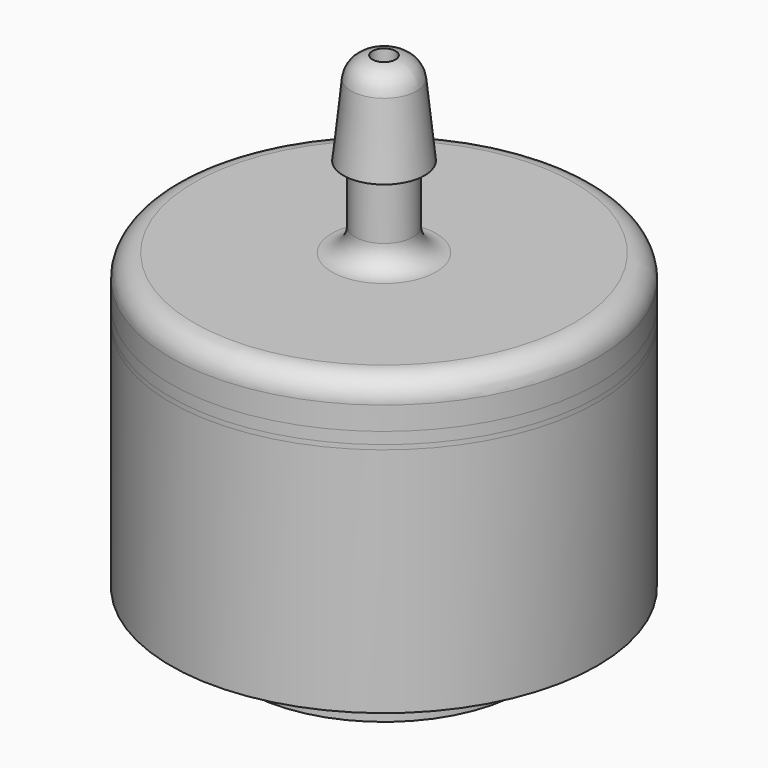
from build123d import *

# Parameters (mm, degrees)
F0_R      = 6
F0_R_2    = 3.1
F0_R_3    = 0.5
F1_DEPTH  = 2
F2_R      = 2.75
F3_DEPTH  = 0.2
F4_R      = 3.1
F4_R_2    = 2.7
F5_DEPTH  = 1
F4_R_3    = 6
F6_DEPTH  = 10
F8_R      = 6
F8_R_2    = 0.5
F9_DEPTH  = 0.2
F8_R_3    = 9.2
F8_R_4    = 6.2
F10_DEPTH = 10
F11_DEPTH = 0.2
F12_R     = 9.2
F12_R_2   = 6.2
F13_DEPTH = 0.5
F14_R     = 9.2
F15_DEPTH = 2
F16_R     = 1.25
F17_DEPTH = 3.5
F18_R     = 1.75
F18_R_2   = 1.25
F19_DEPTH = 4
F19_TAPER = 6
F20_R     = 0.5
F21_DEPTH = 25
F23_R     = 0.5


# Not quite as in the source:
# - a fillet or chamfer that OpenCascade refuses, or shapes differently, is made with other operations: its cross-section is extruded or revolved along the edge and cut away or added
# - a feature names something its author has since deleted; it is built from what else it names


with BuildPart() as f1:
    # F0 (on Top) → F1 (new body)
    with BuildSketch(Plane.XY):
        Circle(F0_R)
        Circle(F0_R_2, mode=Mode.SUBTRACT)
        Circle(F0_R_2)
        with Locations((-1.7320508076, -1)):
            Circle(F0_R_3, mode=Mode.SUBTRACT)
        with Locations((0, -2)):
            Circle(F0_R_3, mode=Mode.SUBTRACT)
        with Locations((1.7320508076, -1)):
            Circle(F0_R_3, mode=Mode.SUBTRACT)
        with Locations((-1.7320508076, 1)):
            Circle(F0_R_3, mode=Mode.SUBTRACT)
        Circle(F0_R_3, mode=Mode.SUBTRACT)
        with Locations((1.7320508076, 1)):
            Circle(F0_R_3, mode=Mode.SUBTRACT)
        with Locations((0, 2)):
            Circle(F0_R_3, mode=Mode.SUBTRACT)
    extrude(amount=-F1_DEPTH)

    # F2 (on face) → F3 (cut)
    with BuildSketch(Plane.XY):
        Circle(F2_R)
        with BuildLine():
            ThreePointArc((2.1364027102, 0.7058919606), (2.221419152, 0.3574869943), (2.25, 0))
            ThreePointArc((2.25, 0), (2.221419152, -0.3574869943), (2.1364027102, -0.7058919606))
            ThreePointArc((2.1364027102, -0.7058919606), (2.2075379006, -0.845364867), (2.2320508076, -1))
            ThreePointArc((2.2320508076, -1), (2.0665171428, -1.3716615), (1.6795217253, -1.4972330394))
            ThreePointArc((1.6795217253, -1.4972330394), (1.125, -1.9485571585), (0.4568809849, -2.203125))
            ThreePointArc((0.4568809849, -2.203125), (0, -2.5), (-0.4568809849, -2.203125))
            ThreePointArc((-0.4568809849, -2.203125), (-1.125, -1.9485571585), (-1.6795217253, -1.4972330394))
            ThreePointArc((-1.6795217253, -1.4972330394), (-2.1650635095, -1.25), (-2.1364027102, -0.7058919606))
            ThreePointArc((-2.1364027102, -0.7058919606), (-2.25, 0), (-2.1364027102, 0.7058919606))
            ThreePointArc((-2.1364027102, 0.7058919606), (-2.1650635095, 1.25), (-1.6795217253, 1.4972330394))
            ThreePointArc((-1.6795217253, 1.4972330394), (-1.125, 1.9485571585), (-0.4568809849, 2.203125))
            ThreePointArc((-0.4568809849, 2.203125), (0, 2.5), (0.4568809849, 2.203125))
            ThreePointArc((0.4568809849, 2.203125), (1.125, 1.9485571585), (1.6795217253, 1.4972330394))
            ThreePointArc((1.6795217253, 1.4972330394), (2.0665171428, 1.3716615), (2.2320508076, 1))
            ThreePointArc((2.2320508076, 1), (2.2075379006, 0.845364867), (2.1364027102, 0.7058919606))
        make_face(mode=Mode.SUBTRACT)
    extrude(amount=-F3_DEPTH, mode=Mode.SUBTRACT)

    # F4 (on face) → F5 (join)
    with BuildSketch(Plane(origin=(0, 0, -2), x_dir=(1, 0, 0), z_dir=(0, 0, -1))):
        Circle(F4_R)
        Circle(F4_R_2, mode=Mode.SUBTRACT)
    extrude(amount=F5_DEPTH)

    # F4 (on face) → F6 (join)
    with BuildSketch(Plane(origin=(0, 0, -2), x_dir=(1, 0, 0), z_dir=(0, 0, -1))):
        Circle(F4_R_3)
        Circle(F4_R, mode=Mode.SUBTRACT)
    extrude(amount=F6_DEPTH)

    # F23
    f23_edges = [f1.edges().sort_by_distance(p)[0] for p in [
        (-6, 0, 0),
    ]]
    fillet(f23_edges, radius=F23_R)


with BuildPart() as f9:
    # F8 (on offset) → F9 (new body)
    with BuildSketch(Plane.XY):
        Circle(F8_R)
        with Locations((-1.7320508076, -1)):
            Circle(F8_R_2, mode=Mode.SUBTRACT)
        with Locations((0, -2)):
            Circle(F8_R_2, mode=Mode.SUBTRACT)
        with Locations((1.7320508076, -1)):
            Circle(F8_R_2, mode=Mode.SUBTRACT)
        with Locations((-1.7320508076, 1)):
            Circle(F8_R_2, mode=Mode.SUBTRACT)
        Circle(F8_R_2, mode=Mode.SUBTRACT)
        with Locations((1.7320508076, 1)):
            Circle(F8_R_2, mode=Mode.SUBTRACT)
        with Locations((0, 2)):
            Circle(F8_R_2, mode=Mode.SUBTRACT)
        with Locations((-1.7320508076, 1)):
            Circle(F8_R_2)
        with Locations((0, 2)):
            Circle(F8_R_2)
        with Locations((1.7320508076, 1)):
            Circle(F8_R_2)
        with Locations((1.7320508076, -1)):
            Circle(F8_R_2)
        with Locations((0, -2)):
            Circle(F8_R_2)
        with Locations((-1.7320508076, -1)):
            Circle(F8_R_2)
        Circle(F8_R_2)
    extrude(amount=F9_DEPTH)


with BuildPart() as f10:
    # F8 (on offset) → F10 (new body)
    with BuildSketch(Plane.XY):
        Circle(F8_R_3)
        Circle(F8_R_4, mode=Mode.SUBTRACT)
    extrude(amount=-F10_DEPTH)

    # F11 (add): a face of the model
    f11_faces = [f10.faces().sort_by_distance(p)[0] for p in [
        (-8.9397847045, 0, 0),
    ]]
    extrude(f11_faces, amount=F11_DEPTH)

    # F12 (on face) → F13 (join)
    with BuildSketch(Plane.XY.offset(0.2)):
        Circle(F12_R)
        Circle(F12_R_2, mode=Mode.SUBTRACT)
        Circle(F12_R_2)
        with BuildLine():
            ThreePointArc((-3, 0), (-2.7071067812, 0.7071067812), (-2, 1))
            Line((-2, 1), (-1, 1))
            Line((-1, 1), (-1, 2))
            ThreePointArc((-1, 2), (-0.7071067812, 2.7071067812), (0, 3))
            ThreePointArc((0, 3), (0.7071067812, 2.7071067812), (1, 2))
            Line((1, 2), (1, 1))
            Line((1, 1), (2, 1))
            ThreePointArc((2, 1), (2.7071067812, 0.7071067812), (3, 0))
            ThreePointArc((3, 0), (2.7071067812, -0.7071067812), (2, -1))
            Line((2, -1), (1, -1))
            Line((1, -1), (1, -2))
            ThreePointArc((1, -2), (0.7071067812, -2.7071067812), (0, -3))
            ThreePointArc((0, -3), (-0.7071067812, -2.7071067812), (-1, -2))
            Line((-1, -2), (-1, -1))
            Line((-1, -1), (-2, -1))
            ThreePointArc((-2, -1), (-2.7071067812, -0.7071067812), (-3, 0))
        make_face(mode=Mode.SUBTRACT)
    extrude(amount=F13_DEPTH)

    # F14 (on face) → F15 (join)
    with BuildSketch(Plane.XY.offset(0.7)):
        Circle(F14_R)
        with BuildLine():
            ThreePointArc((1, -2), (0, -3), (-1, -2))
            Line((-1, -2), (-1, -1))
            Line((-1, -1), (-2, -1))
            ThreePointArc((-2, -1), (-3, 0), (-2, 1))
            Line((-2, 1), (-1, 1))
            Line((-1, 1), (-1, 2))
            ThreePointArc((-1, 2), (0, 3), (1, 2))
            Line((1, 2), (1, 1))
            Line((1, 1), (2, 1))
            ThreePointArc((2, 1), (3, 0), (2, -1))
            Line((2, -1), (1, -1))
            Line((1, -1), (1, -2))
        make_face(mode=Mode.SUBTRACT)
        with BuildLine():
            Line((-1, -1), (-1, -2))
            ThreePointArc((-1, -2), (0, -3), (1, -2))
            Line((1, -2), (1, -1))
            Line((1, -1), (2, -1))
            ThreePointArc((2, -1), (3, 0), (2, 1))
            Line((2, 1), (1, 1))
            Line((1, 1), (1, 2))
            ThreePointArc((1, 2), (0, 3), (-1, 2))
            Line((-1, 2), (-1, 1))
            Line((-1, 1), (-2, 1))
            ThreePointArc((-2, 1), (-3, 0), (-2, -1))
            Line((-2, -1), (-1, -1))
        make_face()
    extrude(amount=F15_DEPTH)

    # F16 (on face) → F17 (join)
    with BuildSketch(Plane.XY.offset(2.7)):
        Circle(F16_R)
    extrude(amount=F17_DEPTH)

    # F18 (on face) → F19 (join)
    with BuildSketch(Plane.XY.offset(6.2)):
        Circle(F18_R)
        Circle(F18_R_2, mode=Mode.SUBTRACT)
        Circle(F18_R_2)
    extrude(amount=F19_DEPTH, taper=F19_TAPER)

    # F20 (on face) → F21 (cut)
    with BuildSketch(Plane.XY.offset(10.2)):
        Circle(F20_R)
    extrude(amount=-F21_DEPTH, mode=Mode.SUBTRACT)

    # F22: fillet of radius 1 on 3 edges, made by hand

    # F22_s1 → F22_t2 (revolve)
    with BuildSketch(Plane.XZ):
        with BuildLine():
            ThreePointArc((1.25, 3.7), (1.5428932188, 2.9928932188), (2.25, 2.7))
            Line((2.25, 2.7), (1.25, 2.7))
            Line((1.25, 2.7), (1.25, 3.7))
        make_face()
    revolve(axis=Axis((0, 0, 2.7), (0, 0, 1)))

    # F22_s3 → F22_t4 (revolve, cut)
    with BuildSketch(Plane.XZ):
        with BuildLine():
            ThreePointArc((1.4234350097, 9.3070583361), (1.1240510304, 9.9214062722), (0.5, 10.2))
            Line((0.5, 10.2), (1.3295830589, 10.2))
            Line((1.3295830589, 10.2), (1.4234350097, 9.3070583361))
        make_face()
    revolve(axis=Axis((0, 0, 10.2), (0, 0, -1)), mode=Mode.SUBTRACT)

    # F22_s5 → F22_t6 (revolve, cut)
    with BuildSketch(Plane.XZ):
        with BuildLine():
            ThreePointArc((8.2, 2.7), (8.9071067812, 2.4071067812), (9.2, 1.7))
            Line((9.2, 1.7), (9.2, 2.7))
            Line((9.2, 2.7), (8.2, 2.7))
        make_face()
    revolve(axis=Axis((0, 0, 2.7), (0, 0, 1)), mode=Mode.SUBTRACT)


solid = Compound([f1.part, f9.part, f10.part])
